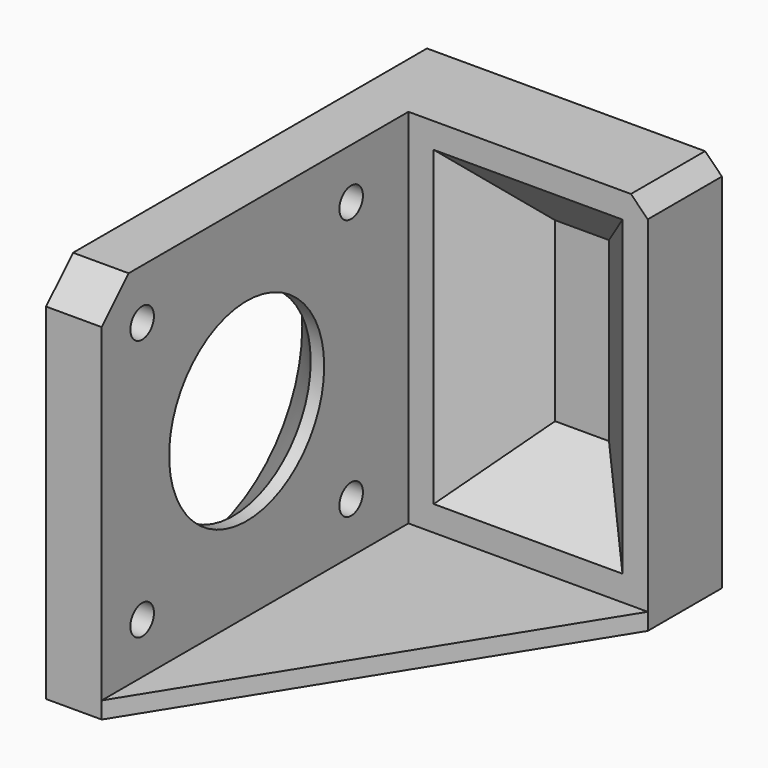
from build123d import *

# Parameters (mm, degrees)
F0_W      = 45.5
F0_H      = 2
F1_DEPTH  = 35
F0_H_2    = 43
F0_R      = 1.75
F0_R_2    = 11.5
F2_DEPTH  = 6.6
F0_W_2    = 6.35
F0_H_3    = 8.8
F3_DEPTH  = 6.6
F4_R      = 2
F5_DEPTH  = 14
F6_W      = 5
F6_H      = 8.3
F7_DEPTH  = 8.39
F8_SIZE2  = 28.4
F8_SIZE   = 45.5
F9_R      = 2
F10_SIZE  = 1
F11_SIZE  = 4
F12_SIZE  = 5
F13_W     = 22.4
F13_H     = 37
F14_DEPTH = 8
F15_SIZE  = 7.99999
F16_SIZE  = 2


# Not quite as in the source:
# - a fillet or chamfer is up to 0.001 mm smaller than in the source, because OpenCascade refuses the exact size


with BuildPart() as f1:
    # F0 (on Right) → F1 (new body)
    with BuildSketch(Plane.YZ):
        Polygon((35, 21.5), (24, 21.5), (24, -21.5), (24, -23.5), (35, -23.5), (35, -17.88), (35, -9.08), (35, 5.92), (35, 14.72), align=None)
        with Locations((1.25, -22.5)):
            Rectangle(F0_W, F0_H)
    extrude(amount=F1_DEPTH)

    # F0 (on Right) → F2 (join)
    with BuildSketch(Plane.YZ):
        with Locations((1.25, 0)):
            Rectangle(F0_W, F0_H_2)
        with Locations((-15.5, -15.5)):
            Circle(F0_R, mode=Mode.SUBTRACT)
        with Locations((15.5, -15.5)):
            Circle(F0_R, mode=Mode.SUBTRACT)
        Circle(F0_R_2, mode=Mode.SUBTRACT)
        with Locations((-15.5, 15.5)):
            Circle(F0_R, mode=Mode.SUBTRACT)
        with Locations((15.5, 15.5)):
            Circle(F0_R, mode=Mode.SUBTRACT)
    extrude(amount=F2_DEPTH)

    # F0 (on Right) → F3 (join)
    with BuildSketch(Plane.YZ):
        with Locations((38.175, 10.32)):
            Rectangle(F0_W_2, F0_H_3)
        with Locations((38.175, -13.48)):
            Rectangle(F0_W_2, F0_H_3)
    extrude(amount=F3_DEPTH)

    # F4 (on face) → F5 (cut)
    with BuildSketch(Plane(origin=(0, 35, 0), x_dir=(-1, 0, 0), z_dir=(0, 1, 0))):
        with Locations((-3.3, -1.58)):
            Circle(F4_R)
    extrude(amount=-F5_DEPTH, mode=Mode.SUBTRACT)

    # F6 (on face) → F7 (cut)
    with BuildSketch(Plane(origin=(0, 0, 0), x_dir=(0, -1, 0), z_dir=(-1, 0, 0))):
        with Locations((-27.5, -1.58)):
            Rectangle(F6_W, F6_H)
    extrude(amount=-F7_DEPTH, mode=Mode.SUBTRACT)

    # F8
    f8_edges = [f1.edges().sort_by_distance(p)[0] for p in [
        (35, -21.5, -22.5),
    ]]
    f8_side = f1.faces().sort_by_distance((35, 25.113055, -4.338737))[0]
    chamfer(f8_edges, length=F8_SIZE, length2=F8_SIZE2, reference=f8_side)

    # F9
    f9_edges = [f1.edges().sort_by_distance(p)[0] for p in [
        (3.3, 41.35, 14.72),
        (3.3, 41.35, 5.92),
        (3.3, 41.35, -9.08),
        (3.3, 41.35, -17.88),
    ]]
    fillet(f9_edges, radius=F9_R)

    # F10
    f10_edges = [f1.edges().sort_by_distance(p)[0] for p in [
        (0, 37.175, -9.08),
        (0, 37.175, 14.72),
        (6.6, 37.175, -17.88),
        (6.6, 37.175, 5.92),
    ]]
    chamfer(f10_edges, length=F10_SIZE)

    # F11
    f11_edges = [f1.edges().sort_by_distance(p)[0] for p in [
        (3.3, -21.5, 21.5),
    ]]
    chamfer(f11_edges, length=F11_SIZE)

    # F12
    f12_edges = [f1.edges().sort_by_distance(p)[0] for p in [
        (0, -11.5, 0),
    ]]
    chamfer(f12_edges, length=F12_SIZE)

    # F13 (on face) → F14 (cut)
    with BuildSketch(Plane.XZ.offset(-24)):
        with Locations((20.8, 0)):
            Rectangle(F13_W, F13_H)
    extrude(amount=-F14_DEPTH, mode=Mode.SUBTRACT)

    # F15 (size 8 in the source; OpenCascade refuses exactly that, so slightly less here)
    f15_edges = [f1.edges().sort_by_distance(p)[0] for p in [
        (20.8, 32, 18.5),
        (9.6, 32, 0),
        (20.8, 32, -18.5),
        (32, 32, 0),
    ]]
    chamfer(f15_edges, length=F15_SIZE)

    # F16
    f16_edges = [f1.edges().sort_by_distance(p)[0] for p in [
        (35, 29.5, 21.5),
    ]]
    chamfer(f16_edges, length=F16_SIZE)


solid = f1.part
